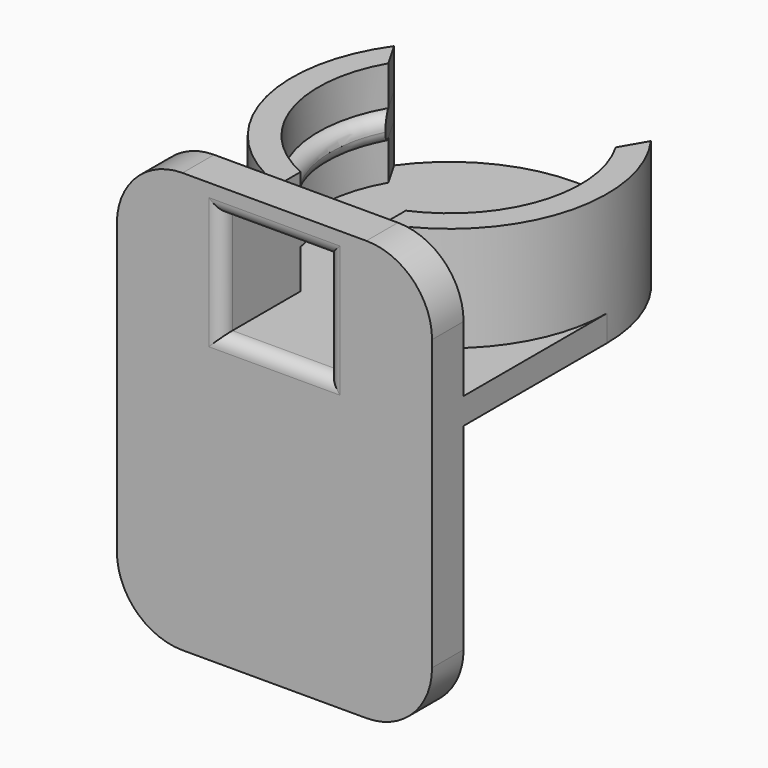
from build123d import *

# Parameters (mm, degrees)
F1_DEPTH  = 2
F3_DEPTH  = 3
F5_DEPTH  = 2
F7_DEPTH  = 3
F8_R      = 0.99999
F9_W      = 24
F9_H      = 22.6653645039
F10_DEPTH = 10
F11_W     = 24
F11_H     = 32
F11_W_2   = 8
F11_H_2   = 8
F12_DEPTH = 3
F13_R     = 1
F14_R     = 5
F15_W     = 24
F15_H     = 13.6653645039
F16_DEPTH = 2


# Not quite as in the source:
# - a fillet or chamfer is up to 0.001 mm smaller than in the source, because OpenCascade refuses the exact size


with BuildPart() as f1:
    # F0 (on Top) → F1 (new body)
    with BuildSketch(Plane.XY):
        with BuildLine():
            ThreePointArc((5.5, 1.5), (0, 24.1653645039), (-5.5, 1.5))
            Line((-5.5, 1.5), (-5.5, -1.5))
            ThreePointArc((-5.5, -1.5), (0, -24.1653645039), (5.5, -1.5))
            Line((5.5, -1.5), (5.5, 1.5))
        make_face()
    extrude(amount=F1_DEPTH)

    # F2 (on face) → F3 (join)
    with BuildSketch(Plane.XY.offset(2)):
        with BuildLine():
            Line((9.7844830762, 19.1125863177), (8.6602540378, 17.1653645039))
            ThreePointArc((8.6602540378, 17.1653645039), (9.4991255677, 9.0402063559), (4, 3.0002131139))
            Line((4, 3.0002131139), (4, -6.2432010007))
            Line((4, -6.2432010007), (9.1651513899, -16.1653645039))
            ThreePointArc((9.1651513899, -16.1653645039), (9.5868378212, -9.3206253964), (5.5, -3.8137179596))
            Line((5.5, -3.8137179596), (5.5, 1.5))
            ThreePointArc((5.5, 1.5), (11.6599594736, 9.3289327537), (9.7844830762, 19.1125863177))
        make_face()
        with BuildLine():
            ThreePointArc((-4, 3.0002131139), (-9.4991255677, 9.0402063559), (-8.6602540378, 17.1653645039))
            Line((-8.6602540378, 17.1653645039), (-9.7844830762, 19.1125863177))
            ThreePointArc((-9.7844830762, 19.1125863177), (-11.6599594736, 9.3289327537), (-5.5, 1.5))
            Line((-5.5, 1.5), (-5.5, -3.8137179596))
            ThreePointArc((-5.5, -3.8137179596), (-9.5868378212, -9.3206253964), (-9.1651513899, -16.1653645039))
            Line((-9.1651513899, -16.1653645039), (-4, -6.2432010007))
            Line((-4, -6.2432010007), (-4, 3.0002131139))
        make_face()
    extrude(amount=F3_DEPTH)

    # F4 (on face) → F5 (join)
    with BuildSketch(Plane.XY.offset(5)):
        with BuildLine():
            Line((-8.0717844057, 16.1461052023), (-9.7844830762, 19.1125863177))
            ThreePointArc((-9.7844830762, 19.1125863177), (-11.6599594736, 9.3289327537), (-5.5, 1.5))
            Line((-5.5, 1.5), (-5.5, -5.0414610795))
            ThreePointArc((-5.5, -5.0414610795), (-8.6043935433, -9.5263473097), (-8.5483759414, -14.980549891))
            Line((-8.5483759414, -14.980549891), (-4, -6.2432010007))
            Line((-4, -6.2432010007), (-4, 4.1031067556))
            ThreePointArc((-4, 4.1031067556), (-8.5258693153, 9.2827350759), (-8.0717844057, 16.1461052023))
        make_face()
        with BuildLine():
            ThreePointArc((5.5, 1.5), (11.6599594736, 9.3289327537), (9.7844830762, 19.1125863177))
            Line((9.7844830762, 19.1125863177), (8.0717844057, 16.1461052023))
            ThreePointArc((8.0717844057, 16.1461052023), (8.5258693153, 9.2827350759), (4, 4.1031067556))
            Line((4, 4.1031067556), (4, -6.2432010007))
            Line((4, -6.2432010007), (8.5483759414, -14.980549891))
            ThreePointArc((8.5483759414, -14.980549891), (8.6043935433, -9.5263473097), (5.5, -5.0414610795))
            Line((5.5, -5.0414610795), (5.5, 1.5))
        make_face()
    extrude(amount=F5_DEPTH)

    # F6 (on face) → F7 (join)
    with BuildSketch(Plane.XY.offset(7)):
        with BuildLine():
            Line((9.7844830762, 19.1125863177), (8.6602540378, 17.1653645039))
            ThreePointArc((8.6602540378, 17.1653645039), (9.4991255677, 9.0402063559), (4, 3.0002131139))
            Line((4, 3.0002131139), (4, -6.2432010007))
            Line((4, -6.2432010007), (9.1651513899, -16.1653645039))
            ThreePointArc((9.1651513899, -16.1653645039), (9.5868378212, -9.3206253964), (5.5, -3.8137179596))
            Line((5.5, -3.8137179596), (5.5, 1.5))
            ThreePointArc((5.5, 1.5), (11.6599594736, 9.3289327537), (9.7844830762, 19.1125863177))
        make_face()
        with BuildLine():
            ThreePointArc((-4, 3.0002131139), (-9.4991255677, 9.0402063559), (-8.6602540378, 17.1653645039))
            Line((-8.6602540378, 17.1653645039), (-9.7844830762, 19.1125863177))
            ThreePointArc((-9.7844830762, 19.1125863177), (-11.6599594736, 9.3289327537), (-5.5, 1.5))
            Line((-5.5, 1.5), (-5.5, -3.8137179596))
            ThreePointArc((-5.5, -3.8137179596), (-9.5868378212, -9.3206253964), (-9.1651513899, -16.1653645039))
            Line((-9.1651513899, -16.1653645039), (-4, -6.2432010007))
            Line((-4, -6.2432010007), (-4, 3.0002131139))
        make_face()
    extrude(amount=F7_DEPTH)

    # F8 (radius 1 in the source; OpenCascade refuses exactly that, so slightly less here)
    f8_edges = [f1.edges().sort_by_distance(p)[0] for p in [
        (8.525869, 9.282735, 7),
        (-8.525869, 9.282735, 7),
        (-8.525869, 9.282735, 5),
        (8.525869, 9.282735, 5),
        (-8.604394, -9.526347, 5),
        (-8.604394, -9.526347, 7),
        (8.604394, -9.526347, 7),
        (8.604394, -9.526347, 5),
    ]]
    fillet(f8_edges, radius=F8_R)

    # F9 (on face) → F10 (cut)
    with BuildSketch(Plane.XY.offset(10)):
        with Locations((0, -12.8326822519)):
            Rectangle(F9_W, F9_H)
    extrude(amount=-F10_DEPTH, mode=Mode.SUBTRACT)

    # F11 (on face) → F12 (join)
    with BuildSketch(Plane.XZ.offset(1.5)):
        with Locations((0, -4)):
            Rectangle(F11_W, F11_H)
        with Locations((0, 6)):
            Rectangle(F11_W_2, F11_H_2, mode=Mode.SUBTRACT)
    extrude(amount=F12_DEPTH)

    # F13
    f13_edges = [f1.edges().sort_by_distance(p)[0] for p in [
        (0, -4.5, 10),
        (4, -4.5, 6),
        (-4, -4.5, 6),
        (0, -4.5, 2),
    ]]
    fillet(f13_edges, radius=F13_R)

    # F14
    f14_edges = [f1.edges().sort_by_distance(p)[0] for p in [
        (-12, -3, 12),
        (12, -3, 12),
        (12, -3, -20),
        (-12, -3, -20),
    ]]
    fillet(f14_edges, radius=F14_R)

    # F15 (on face) → F16 (join)
    with BuildSketch(Plane(origin=(0, 0, 0), x_dir=(1, 0, 0), z_dir=(0, 0, -1))):
        with Locations((0, -5.3326822519)):
            Rectangle(F15_W, F15_H)
    extrude(amount=-F16_DEPTH)


solid = f1.part
